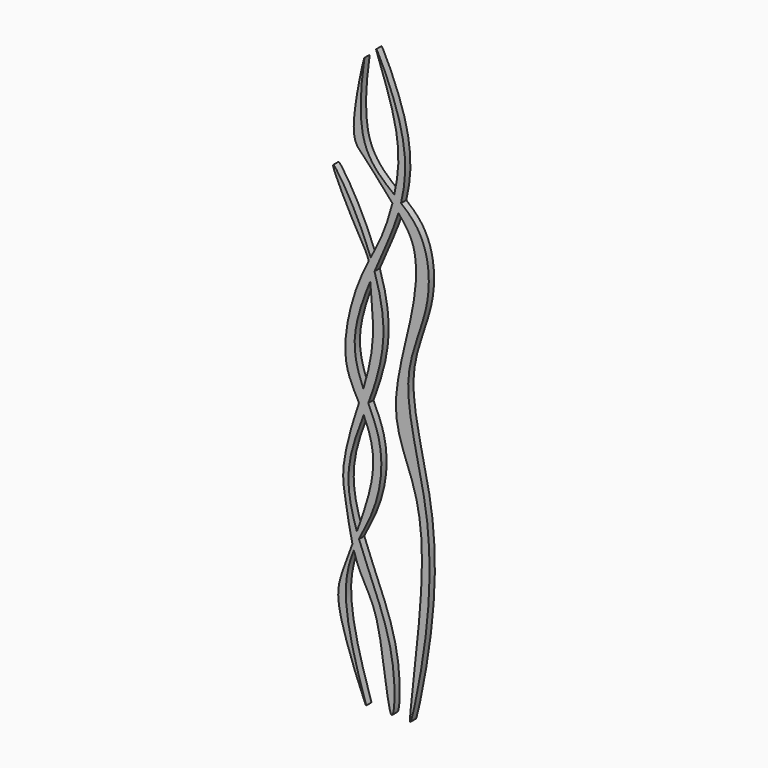
from build123d import *

# Parameters (mm, degrees)
F1_DEPTH = 5


with BuildPart() as f1:
    # F0 (on Front) → F1 (new body)
    with BuildSketch(Plane.XZ):
        with BuildLine():
            Line((35.8674378101, 431.1320186524), (35.8513072133, 431.1164320212))
            add(Edge.make_bspline(
                [(57.0998449271, 341.0998456277), (49.9220262035, 349.1582779695), (35.7068085968, 365.9917878999), (22.6830832762, 375.8339488035), (35.1904588041, 430.2411726906), (35.8513072133, 431.1164320212)],
                knots=[0.8554541645, 0.8554541645, 0.8554541645, 0.8554541645, 0.9033771043, 0.9393274439, 1, 1, 1, 1], degree=3))
            add(Edge.make_bspline(
                [(58.5453930095, 347.3112772335), (58.1063605359, 345.2660695194), (57.6239104858, 343.1895858755), (57.0998449271, 341.0998456277)],
                knots=[0.5531351189, 0.5531351189, 0.5531351189, 0.5531351189, 0.5610706359, 0.5610706359, 0.5610706359, 0.5610706359], degree=3))
            add(Edge.make_bspline(
                [(35.8674378101, 431.1320186524), (36.4193802026, 431.4208404043), (25.0122183986, 374.254364866), (49.3355566618, 354.5325447132), (58.5453930096, 347.3112772335)],
                knots=[0.0005468821, 0.0005468821, 0.0005468821, 0.0005468821, 0.0634099902, 0.1031710958, 0.1031710958, 0.1031710958, 0.1031710958], degree=3))
        make_face()
        with BuildLine():
            add(Edge.make_bspline(
                [(12.2896667845, 352.1445277356), (13.8353158875, 352.8439195348), (29.9358109145, 328.3983784934), (40.6642300023, 299.6400147025)],
                knots=[0, 0, 0, 0, 0.0674576457, 0.0674576457, 0.0674576457, 0.0674576457], degree=3))
            Line((12.2896667845, 352.1445277356), (12.2552961627, 351.1596819636))
            add(Edge.make_bspline(
                [(39.1945759637, 296.7898729903), (37.7226031359, 302.1994928843), (29.3261172958, 314.5522785171), (13.2198845893, 346.9232672187), (12.2552961627, 351.1596819636)],
                knots=[0.8926549531, 0.8926549531, 0.8926549531, 0.8926549531, 0.9409827893, 0.9930061016, 0.9930061016, 0.9930061016, 0.9930061016], degree=3))
            add(Edge.make_bspline(
                [(40.6642300023, 299.6400147025), (40.1711501967, 298.6874374799), (39.68057784, 297.7380475246), (39.1945759637, 296.7898729903)],
                knots=[0.6176191477, 0.6176191477, 0.6176191477, 0.6176191477, 0.6219873359, 0.6219873359, 0.6219873359, 0.6219873359], degree=3))
        make_face()
        with BuildLine():
            add(Edge.make_bspline(
                [(61.5880377942, 336.050528311), (60.1532886926, 337.6950445129), (58.6485487605, 339.3611384328), (57.0998449271, 341.0998456277)],
                knots=[0.8451141931, 0.8451141931, 0.8451141931, 0.8451141931, 0.8554541645, 0.8554541645, 0.8554541645, 0.8554541645], degree=3))
            add(Edge.make_bspline(
                [(57.0998449271, 341.0998456277), (55.2028371849, 333.5354228882), (50.3948878666, 318.3019799337), (43.80494974, 305.7075478904), (40.6642300023, 299.6400147025)],
                knots=[0.5610706359, 0.5610706359, 0.5610706359, 0.5610706359, 0.5897955481, 0.6176191477, 0.6176191477, 0.6176191477, 0.6176191477], degree=3))
            add(Edge.make_bspline(
                [(40.6642300023, 299.6400147025), (41.6822733929, 296.9110700235), (42.6519437571, 294.1432903966), (43.5562143395, 291.3544760241)],
                knots=[0.0674576457, 0.0674576457, 0.0674576457, 0.0674576457, 0.0738588508, 0.0738588508, 0.0738588508, 0.0738588508], degree=3))
            add(Edge.make_bspline(
                [(43.5562143395, 291.3544760241), (49.3562773152, 304.885406405), (56.5094222234, 320.3303584097), (61.0548414458, 334.3038817543), (61.5880377942, 336.050528311)],
                knots=[0.2788743971, 0.2788743971, 0.2788743971, 0.2788743971, 0.310184807, 0.3147174332, 0.3147174332, 0.3147174332, 0.3147174332], degree=3))
        make_face()
        with BuildLine():
            add(Edge.make_bspline(
                [(58.5453930095, 347.3112772335), (58.1063605359, 345.2660695194), (57.6239104858, 343.1895858755), (57.0998449271, 341.0998456277)],
                knots=[0.5531351189, 0.5531351189, 0.5531351189, 0.5531351189, 0.5610706359, 0.5610706359, 0.5610706359, 0.5610706359], degree=3))
            add(Edge.make_bspline(
                [(61.5880377942, 336.050528311), (60.1532886926, 337.6950445129), (58.6485487605, 339.3611384328), (57.0998449271, 341.0998456277)],
                knots=[0.8451141931, 0.8451141931, 0.8451141931, 0.8451141931, 0.8554541645, 0.8554541645, 0.8554541645, 0.8554541645], degree=3))
            add(Edge.make_bspline(
                [(61.5880377942, 336.050528311), (62.3390610706, 338.5107331184), (63.0075384229, 340.9304406114), (63.593734914, 343.3183639912)],
                knots=[0.3147174332, 0.3147174332, 0.3147174332, 0.3147174332, 0.321101775, 0.321101775, 0.321101775, 0.321101775], degree=3))
            add(Edge.make_bspline(
                [(58.5453930096, 347.3112772335), (60.2472141901, 345.9769097721), (61.9417253898, 344.6568772216), (63.593734914, 343.3183639912)],
                knots=[0.1031710958, 0.1031710958, 0.1031710958, 0.1031710958, 0.1105182721, 0.1105182721, 0.1105182721, 0.1105182721], degree=3))
        make_face()
        with BuildLine():
            add(Edge.make_bspline(
                [(40.6642300023, 299.6400147025), (41.6822733929, 296.9110700235), (42.6519437571, 294.1432903966), (43.5562143395, 291.3544760241)],
                knots=[0.0674576457, 0.0674576457, 0.0674576457, 0.0674576457, 0.0738588508, 0.0738588508, 0.0738588508, 0.0738588508], degree=3))
            add(Edge.make_bspline(
                [(40.6642300023, 299.6400147025), (40.1711501967, 298.6874374799), (39.68057784, 297.7380475246), (39.1945759637, 296.7898729903)],
                knots=[0.6176191477, 0.6176191477, 0.6176191477, 0.6176191477, 0.6219873359, 0.6219873359, 0.6219873359, 0.6219873359], degree=3))
            add(Edge.make_bspline(
                [(40.2937896927, 283.5921728742), (39.9715085024, 289.1582650698), (40.2721932454, 292.8295418112), (39.1945759637, 296.7898729903)],
                knots=[0.8572746048, 0.8572746048, 0.8572746048, 0.8572746048, 0.8926549531, 0.8926549531, 0.8926549531, 0.8926549531], degree=3))
            add(Edge.make_bspline(
                [(40.2937896927, 283.5921728742), (41.3534688284, 286.1759804123), (42.4466343673, 288.7659438963), (43.5562143395, 291.3544760241)],
                knots=[0.2728845649, 0.2728845649, 0.2728845649, 0.2728845649, 0.2788743971, 0.2788743971, 0.2788743971, 0.2788743971], degree=3))
        make_face()
        with BuildLine():
            Line((44.8655476692, 439.826688896), (44.82217557, 439.7847794166))
            add(Edge.make_bspline(
                [(44.82217557, 439.7847794166), (44.5575079971, 439.0140407887), (54.7412858712, 413.2672332545), (62.7592801133, 381.9779381012), (61.4167128454, 361.8627670958), (59.0409555069, 349.6198268359), (58.5453930095, 347.3112772335)],
                knots=[0.4235934199, 0.4235934199, 0.4235934199, 0.4235934199, 0.4589892395, 0.5047974731, 0.544177821, 0.5531351189, 0.5531351189, 0.5531351189, 0.5531351189], degree=3))
            add(Edge.make_bspline(
                [(58.5453930096, 347.3112772335), (60.2472141901, 345.9769097721), (61.9417253898, 344.6568772216), (63.593734914, 343.3183639912)],
                knots=[0.1031710958, 0.1031710958, 0.1031710958, 0.1031710958, 0.1105182721, 0.1105182721, 0.1105182721, 0.1105182721], degree=3))
            add(Edge.make_bspline(
                [(63.593734914, 343.3183639912), (68.3202134335, 362.5720933011), (67.0949023012, 396.3919583489), (45.6960828086, 439.8953876713), (44.8655476692, 439.826688896)],
                knots=[0.321101775, 0.321101775, 0.321101775, 0.321101775, 0.3725784641, 0.4223930955, 0.4223930955, 0.4223930955, 0.4223930955], degree=3))
        make_face()
        with BuildLine():
            add(Edge.make_bspline(
                [(61.5880377942, 336.050528311), (62.3390610706, 338.5107331184), (63.0075384229, 340.9304406114), (63.593734914, 343.3183639912)],
                knots=[0.3147174332, 0.3147174332, 0.3147174332, 0.3147174332, 0.321101775, 0.321101775, 0.321101775, 0.321101775], degree=3))
            add(Edge.make_bspline(
                [(70.5356374383, 0), (69.4127842416, 2.0142912314), (82.4408284229, 94.4723585701), (77.7575008021, 155.8600970407), (51.5667689723, 202.6772299468), (74.3102016089, 271.7146354132), (76.9256762295, 316.772031406), (66.2995752714, 330.6501417844), (61.5880377942, 336.050528311)],
                knots=[0.4725961335, 0.4725961335, 0.4725961335, 0.4725961335, 0.5512465321, 0.6234696062, 0.6822934542, 0.753925831, 0.8111590139, 0.8451141931, 0.8451141931, 0.8451141931, 0.8451141931], degree=3))
            Line((70.5356374383, 0), (70.7314392341, 0))
            add(Edge.make_bspline(
                [(63.593734914, 343.3183639912), (67.3850140373, 340.2465431618), (83.8605319287, 325.6103921197), (88.6445326767, 279.7979791621), (59.0979161723, 227.7674234464), (89.413891187, 142.1465922237), (83.8102024378, 56.6499563651), (71.953813944, 1.3400569333), (70.7314392341, 0)],
                knots=[0.1105182721, 0.1105182721, 0.1105182721, 0.1105182721, 0.1273796738, 0.1883895152, 0.2522414383, 0.3306307575, 0.415645216, 0.4690936869, 0.4690936869, 0.4690936869, 0.4690936869], degree=3))
        make_face()
        with BuildLine():
            add(Edge.make_bspline(
                [(40.2937896927, 283.5921728742), (39.9715085024, 289.1582650698), (40.2721932454, 292.8295418112), (39.1945759637, 296.7898729903)],
                knots=[0.8572746048, 0.8572746048, 0.8572746048, 0.8572746048, 0.8926549531, 0.8926549531, 0.8926549531, 0.8926549531], degree=3))
            add(Edge.make_bspline(
                [(39.1945759637, 296.7898729903), (38.0455155245, 294.5480918365), (32.3010441982, 283.1206895811), (24.097701311, 260.6917340732), (18.584574908, 224.1147001091), (28.0975780771, 206.834966316), (31.8096576485, 199.8881902095)],
                knots=[0.6219873359, 0.6219873359, 0.6219873359, 0.6219873359, 0.6323150991, 0.6747927911, 0.7212550824, 0.7533231229, 0.7533231229, 0.7533231229, 0.7533231229], degree=3))
            add(Edge.make_bspline(
                [(31.8096576485, 199.8881902095), (32.9241676637, 203.3444800257), (34.0418040091, 206.8495756675), (35.1100143168, 210.3870609112)],
                knots=[0.7400845811, 0.7400845811, 0.7400845811, 0.7400845811, 0.7539995052, 0.7539995052, 0.7539995052, 0.7539995052], degree=3))
            add(Edge.make_bspline(
                [(35.1100143168, 210.3870609112), (31.513103002, 218.9771643579), (24.5605282156, 240.1950350225), (33.7207257806, 267.5651213715), (40.2937896927, 283.5921728742)],
                knots=[0.2084829517, 0.2084829517, 0.2084829517, 0.2084829517, 0.2357303469, 0.2728845649, 0.2728845649, 0.2728845649, 0.2728845649], degree=3))
        make_face()
        with BuildLine():
            add(Edge.make_bspline(
                [(43.5562143395, 291.3544760241), (46.6492149136, 281.8155121085), (54.5843733536, 248.4604648707), (45.7116082482, 220.5227424268), (38.7918223454, 202.0127868051)],
                knots=[0.0738588508, 0.0738588508, 0.0738588508, 0.0738588508, 0.0957537695, 0.1484936743, 0.1484936743, 0.1484936743, 0.1484936743], degree=3))
            add(Edge.make_bspline(
                [(40.2937896927, 283.5921728742), (41.3534688284, 286.1759804123), (42.4466343673, 288.7659438963), (43.5562143395, 291.3544760241)],
                knots=[0.2728845649, 0.2728845649, 0.2728845649, 0.2728845649, 0.2788743971, 0.2788743971, 0.2788743971, 0.2788743971], degree=3))
            add(Edge.make_bspline(
                [(35.1100143168, 210.3870609112), (38.1867237885, 220.5758919643), (45.0582931243, 247.5231233255), (40.8694511209, 273.6499712204), (40.2937896927, 283.5921728742)],
                knots=[0.7539995052, 0.7539995052, 0.7539995052, 0.7539995052, 0.7940779229, 0.8572746048, 0.8572746048, 0.8572746048, 0.8572746048], degree=3))
            add(Edge.make_bspline(
                [(38.7918223453, 202.0127868051), (37.5465206798, 204.7793118833), (36.2928320893, 207.5622687118), (35.1100143168, 210.3870609112)],
                knots=[0.1995228467, 0.1995228467, 0.1995228467, 0.1995228467, 0.2084829517, 0.2084829517, 0.2084829517, 0.2084829517], degree=3))
        make_face()
        with BuildLine():
            add(Edge.make_bspline(
                [(26.8193321931, 104.3448436892), (24.2562590636, 97.4186895103), (17.3622436446, 79.0359168944), (11.978106445, 59.359887296), (36.4354359891, 0.3760440682), (37.1853150427, 0)],
                knots=[0.8774090514, 0.8774090514, 0.8774090514, 0.8774090514, 0.9008481554, 0.9430294702, 1, 1, 1, 1], degree=3))
            Line((37.1853150427, 0), (37.2056326614, 0))
            add(Edge.make_bspline(
                [(37.2056326614, 0), (37.6999091708, 0.408537232), (15.6710432353, 58.686258116), (24.1576011734, 91.1328001204), (27.9045119255, 100.3826121198)],
                knots=[0.0006420706, 0.0006420706, 0.0006420706, 0.0006420706, 0.0628122762, 0.0917003268, 0.0917003268, 0.0917003268, 0.0917003268], degree=3))
            add(Edge.make_bspline(
                [(27.9045119255, 100.3826121198), (27.5257852859, 101.6637462284), (27.1642459736, 102.9823118881), (26.8193321931, 104.3448436892)],
                knots=[0.5605032011, 0.5605032011, 0.5605032011, 0.5605032011, 0.5687109224, 0.5687109224, 0.5687109224, 0.5687109224], degree=3))
        make_face()
        with BuildLine():
            add(Edge.make_bspline(
                [(31.8096576485, 199.8881902095), (32.9241676637, 203.3444800257), (34.0418040091, 206.8495756675), (35.1100143168, 210.3870609112)],
                knots=[0.7400845811, 0.7400845811, 0.7400845811, 0.7400845811, 0.7539995052, 0.7539995052, 0.7539995052, 0.7539995052], degree=3))
            add(Edge.make_bspline(
                [(31.8096576485, 199.8881902095), (32.975924201, 197.7056420003), (34.1891906105, 195.412887704), (35.3020524964, 193.0987365733), (35.360505676, 192.9765376361)],
                knots=[0.7533231229, 0.7533231229, 0.7533231229, 0.7533231229, 0.7633983064, 0.7639596935, 0.7639596935, 0.7639596935, 0.7639596935], degree=3))
            add(Edge.make_bspline(
                [(38.7918223454, 202.0127868051), (37.6541483184, 198.9695863295), (36.4989062183, 195.9596854974), (35.360505676, 192.9765376361)],
                knots=[0.1484936743, 0.1484936743, 0.1484936743, 0.1484936743, 0.1571645813, 0.1571645813, 0.1571645813, 0.1571645813], degree=3))
            add(Edge.make_bspline(
                [(38.7918223453, 202.0127868051), (37.5465206798, 204.7793118833), (36.2928320893, 207.5622687118), (35.1100143168, 210.3870609112)],
                knots=[0.1995228467, 0.1995228467, 0.1995228467, 0.1995228467, 0.2084829517, 0.2084829517, 0.2084829517, 0.2084829517], degree=3))
        make_face()
        with BuildLine():
            add(Edge.make_bspline(
                [(31.8096576485, 199.8881902095), (32.975924201, 197.7056420003), (34.1891906105, 195.412887704), (35.3020524964, 193.0987365733), (35.360505676, 192.9765376361)],
                knots=[0.7533231229, 0.7533231229, 0.7533231229, 0.7533231229, 0.7633983064, 0.7639596935, 0.7639596935, 0.7639596935, 0.7639596935], degree=3))
            add(Edge.make_bspline(
                [(26.8193321931, 104.3448436892), (24.7056395596, 112.6946794847), (21.9686916144, 131.0735152042), (18.1346010276, 149.8218970327), (23.9108909008, 175.7115802389), (30.208072729, 194.921396218), (31.8096576485, 199.8881902095)],
                knots=[0.5687109224, 0.5687109224, 0.5687109224, 0.5687109224, 0.6190092893, 0.6611445494, 0.7200884102, 0.7400845811, 0.7400845811, 0.7400845811, 0.7400845811], degree=3))
            add(Edge.make_bspline(
                [(30.2341259635, 113.6643468976), (29.0998202538, 110.5245228934), (27.9497928337, 107.3996705687), (26.8193321931, 104.3448436892)],
                knots=[0.8670710769, 0.8670710769, 0.8670710769, 0.8670710769, 0.8774090514, 0.8774090514, 0.8774090514, 0.8774090514], degree=3))
            add(Edge.make_bspline(
                [(35.360505676, 192.9765376361), (29.6557305601, 178.0273285883), (20.0616706378, 152.0935780151), (26.1501193525, 125.6582340555), (30.2341259635, 113.6643468976)],
                knots=[0.1571645813, 0.1571645813, 0.1571645813, 0.1571645813, 0.2006164004, 0.2360914329, 0.2360914329, 0.2360914329, 0.2360914329], degree=3))
        make_face()
        with BuildLine():
            add(Edge.make_bspline(
                [(31.8319427222, 109.1430054801), (35.0123043245, 115.726071429), (47.0412011465, 137.8967600331), (52.2633437262, 172.0396348357), (41.7838728241, 195.3657366055), (38.7918223453, 202.0127868051)],
                knots=[0.1011100663, 0.1011100663, 0.1011100663, 0.1011100663, 0.1228815286, 0.1779946601, 0.1995228467, 0.1995228467, 0.1995228467, 0.1995228467], degree=3))
            add(Edge.make_bspline(
                [(38.7918223454, 202.0127868051), (37.6541483184, 198.9695863295), (36.4989062183, 195.9596854974), (35.360505676, 192.9765376361)],
                knots=[0.1484936743, 0.1484936743, 0.1484936743, 0.1484936743, 0.1571645813, 0.1571645813, 0.1571645813, 0.1571645813], degree=3))
            add(Edge.make_bspline(
                [(35.360505676, 192.9765376361), (39.4718420005, 184.3816086358), (45.3161447579, 165.2275217961), (39.0294570369, 138.6397661284), (32.2174652197, 119.1543450103), (30.2341259635, 113.6643468976)],
                knots=[0.7639596935, 0.7639596935, 0.7639596935, 0.7639596935, 0.8034451596, 0.8489950765, 0.8670710769, 0.8670710769, 0.8670710769, 0.8670710769], degree=3))
            add(Edge.make_bspline(
                [(30.2341259635, 113.6643468976), (30.746705759, 112.1590054981), (31.2805112667, 110.6518987666), (31.8319427222, 109.1430054801)],
                knots=[0.2360914329, 0.2360914329, 0.2360914329, 0.2360914329, 0.2405438705, 0.2405438705, 0.2405438705, 0.2405438705], degree=3))
        make_face()
        with BuildLine():
            Line((56.5284974873, 0), (56.7415849967, 0))
            add(Edge.make_bspline(
                [(31.8319427222, 109.1430054801), (39.4021342098, 88.4285340841), (61.6670436258, 45.3969807634), (58.8952479256, 0.7290711884), (56.7415849967, 0)],
                knots=[0.2405438705, 0.2405438705, 0.2405438705, 0.2405438705, 0.301668069, 0.365490306, 0.365490306, 0.365490306, 0.365490306], degree=3))
            add(Edge.make_bspline(
                [(27.9045119255, 100.3826121198), (29.1249976759, 103.3955645188), (30.4573738615, 106.2977700659), (31.8319427222, 109.1430054801)],
                knots=[0.0917003268, 0.0917003268, 0.0917003268, 0.0917003268, 0.1011100663, 0.1011100663, 0.1011100663, 0.1011100663], degree=3))
            add(Edge.make_bspline(
                [(56.5284974873, 0), (54.5248132789, 0.6726237143), (49.6869985143, 39.3624492812), (44.3938878522, 67.2010997947), (33.8785459391, 84.1356171322), (29.5476302345, 94.8243685473), (27.9045119255, 100.3826121198)],
                knots=[0.3675738913, 0.3675738913, 0.3675738913, 0.3675738913, 0.4258158014, 0.4820840861, 0.5248937256, 0.5605032011, 0.5605032011, 0.5605032011, 0.5605032011], degree=3))
        make_face()
        with BuildLine():
            add(Edge.make_bspline(
                [(30.2341259635, 113.6643468976), (29.0998202538, 110.5245228934), (27.9497928337, 107.3996705687), (26.8193321931, 104.3448436892)],
                knots=[0.8670710769, 0.8670710769, 0.8670710769, 0.8670710769, 0.8774090514, 0.8774090514, 0.8774090514, 0.8774090514], degree=3))
            add(Edge.make_bspline(
                [(27.9045119255, 100.3826121198), (27.5257852859, 101.6637462284), (27.1642459736, 102.9823118881), (26.8193321931, 104.3448436892)],
                knots=[0.5605032011, 0.5605032011, 0.5605032011, 0.5605032011, 0.5687109224, 0.5687109224, 0.5687109224, 0.5687109224], degree=3))
            add(Edge.make_bspline(
                [(27.9045119255, 100.3826121198), (29.1249976759, 103.3955645188), (30.4573738615, 106.2977700659), (31.8319427222, 109.1430054801)],
                knots=[0.0917003268, 0.0917003268, 0.0917003268, 0.0917003268, 0.1011100663, 0.1011100663, 0.1011100663, 0.1011100663], degree=3))
            add(Edge.make_bspline(
                [(30.2341259635, 113.6643468976), (30.746705759, 112.1590054981), (31.2805112667, 110.6518987666), (31.8319427222, 109.1430054801)],
                knots=[0.2360914329, 0.2360914329, 0.2360914329, 0.2360914329, 0.2405438705, 0.2405438705, 0.2405438705, 0.2405438705], degree=3))
        make_face()
    extrude(amount=F1_DEPTH)


solid = f1.part
